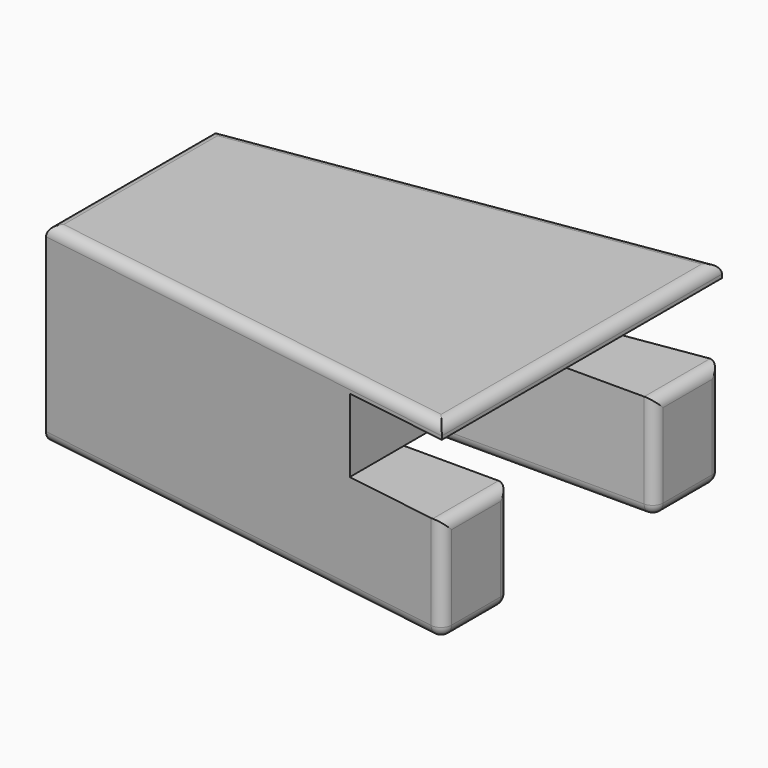
from build123d import *

# Parameters (mm, degrees)
F0_W         = 64.5
F0_H         = 13
F0_H_2       = 2
F1_DEPTH     = 12.5
F2_DEPTH     = 15
F4_DEPTH     = 15
F6_T1_DEPTH  = 72.7705906209
F6_T3_DEPTH  = 57.5
F6_T5_DEPTH  = 72.7705906209
F6_T7_DEPTH  = 37.5
F6_T9_DEPTH  = 66.75
F6_T11_DEPTH = 67.2701117692
F6_T13_DEPTH = 8.7495211484
F6_T15_DEPTH = 67.2701117692
F6_T17_DEPTH = 8.7495211484
F6_T19_DEPTH = 17.8761971291
F6_T21_DEPTH = 17.25
F6_T23_DEPTH = 19.5
F6_T25_DEPTH = 19.5
F6_S29_W     = 1.53
F6_S29_H     = 1.53
F6_T30_DEPTH = 1.53
F6_T36_DEPTH = 1.53
F6_S41_W     = 1.53
F6_S41_H     = 1.53
F6_T42_DEPTH = 1.53
F6_T48_DEPTH = 1.53
F6_T54_DEPTH = 9.5
F6_S55_R     = 1.5
F6_T56_DEPTH = 6
F6_T60_DEPTH = 9.5
F6_S61_R     = 1.5
F6_T62_DEPTH = 6
F6_T66_DEPTH = 9.5
F6_S67_R     = 1.5
F6_T68_DEPTH = 6
F6_T72_DEPTH = 9.5
F6_S73_R     = 1.5
F6_T74_DEPTH = 6


# Not quite as in the source:
# - a fillet or chamfer that OpenCascade refuses, or shapes differently, is made with other operations: its cross-section is extruded or revolved along the edge and cut away or added
# - a feature names something its author has since deleted; it is built from what else it names


with BuildPart() as f1:
    # F0 (on Top) → F1 (new body)
    with BuildSketch(Plane.XY):
        with Locations((-32.25, -6.5)):
            Rectangle(F0_W, F0_H)
        with Locations((-32.25, -14)):
            Rectangle(F0_W, F0_H_2)
        Polygon((0, -15), (-64.5, -15), (0, -25), align=None)
    extrude(amount=F1_DEPTH)

    # F0 (on Top) → F2 (join)
    with BuildSketch(Plane.XY):
        with Locations((-32.25, -14)):
            Rectangle(F0_W, F0_H_2)
        Polygon((0, -15), (-64.5, -15), (0, -25), align=None)
    extrude(amount=-F2_DEPTH)

    # F3 (on face) → F4 (cut)
    with BuildSketch(Plane.YZ):
        Polygon((-13, 0), (0, 0), (0, 10.5), (-25, 10.5), (-25, 0), align=None)
    extrude(amount=-F4_DEPTH, mode=Mode.SUBTRACT)

    # F5: F1 across plane


with BuildPart() as f1_1:
    add(f1.part)
    add(f1.part.mirror(Plane.XZ))

    # F6: fillet of radius 1.5 on 18 edges, made by hand

    # F6_s2 → F6_t1 (cut)
    with BuildSketch(Plane(origin=(-64.4207380098, 9.9877113194, 0), x_dir=(0, 0, 1), z_dir=(0.9881939076, -0.1532083578, 0))):
        with BuildLine():
            ThreePointArc((11, 24.7048476911), (12.0606601718, 24.2655078629), (12.5, 23.2048476911))
            Line((12.5, 23.2048476911), (12.5, 24.7048476911))
            Line((12.5, 24.7048476911), (11, 24.7048476911))
        make_face()
    extrude(amount=F6_T1_DEPTH, mode=Mode.SUBTRACT)

    # F6_s4 → F6_t3 (cut)
    with BuildSketch(Plane.XZ.offset(-28.75)):
        with BuildLine():
            ThreePointArc((-1.5, 12.5), (-0.4393398282, 12.0606601718), (0, 11))
            Line((0, 11), (0, 12.5))
            Line((0, 12.5), (-1.5, 12.5))
        make_face()
    extrude(amount=F6_T3_DEPTH, mode=Mode.SUBTRACT)

    # F6_s6 → F6_t5 (cut)
    with BuildSketch(Plane(origin=(-64.4207380098, -9.9877113194, 0), x_dir=(0, 0, 1), z_dir=(0.9881939076, 0.1532083578, 0))):
        with BuildLine():
            ThreePointArc((12.5, -23.2048476911), (12.0606601718, -24.2655078629), (11, -24.7048476911))
            Line((11, -24.7048476911), (12.5, -24.7048476911))
            Line((12.5, -24.7048476911), (12.5, -23.2048476911))
        make_face()
    extrude(amount=F6_T5_DEPTH, mode=Mode.SUBTRACT)

    # F6_s8 → F6_t7 (cut)
    with BuildSketch(Plane.XZ.offset(-18.75)):
        with BuildLine():
            ThreePointArc((-63, 12.5), (-64.0606601718, 12.0606601718), (-64.5, 11))
            Line((-64.5, 11), (-64.5, 12.5))
            Line((-64.5, 12.5), (-63, 12.5))
        make_face()
    extrude(amount=F6_T7_DEPTH, mode=Mode.SUBTRACT)

    # F6_s10 → F6_t9 (cut)
    with BuildSketch(Plane.YZ.offset(-68.25)):
        with BuildLine():
            ThreePointArc((-13, -13.5), (-13.4393398282, -14.5606601718), (-14.5, -15))
            Line((-14.5, -15), (-13, -15))
            Line((-13, -15), (-13, -13.5))
        make_face()
        with BuildLine():
            ThreePointArc((13, -13.5), (13.4393398282, -14.5606601718), (14.5, -15))
            Line((14.5, -15), (13, -15))
            Line((13, -15), (13, -13.5))
        make_face()
    extrude(amount=F6_T9_DEPTH, mode=Mode.SUBTRACT)

    # F6_s12 → F6_t11 (cut)
    with BuildSketch(Plane(origin=(-64.4207380098, 9.9877113194, 0), x_dir=(0, 0, 1), z_dir=(0.9881939076, -0.1532083578, 0))):
        with BuildLine():
            ThreePointArc((-13.5, 24.7048476911), (-14.5606601718, 24.2655078629), (-15, 23.2048476911))
            Line((-15, 23.2048476911), (-15, 24.7048476911))
            Line((-15, 24.7048476911), (-13.5, 24.7048476911))
        make_face()
    extrude(amount=F6_T11_DEPTH, mode=Mode.SUBTRACT)

    # F6_s14 → F6_t13 (cut)
    with BuildSketch(Plane.XZ.offset(14.5)):
        with BuildLine():
            ThreePointArc((0, -13.5), (-0.4393398282, -14.5606601718), (-1.5, -15))
            Line((-1.5, -15), (0, -15))
            Line((0, -15), (0, -13.5))
        make_face()
    extrude(amount=F6_T13_DEPTH, mode=Mode.SUBTRACT)

    # F6_s16 → F6_t15 (cut)
    with BuildSketch(Plane(origin=(-64.4207380098, -9.9877113194, 0), x_dir=(0, 0, 1), z_dir=(0.9881939076, 0.1532083578, 0))):
        with BuildLine():
            ThreePointArc((-15, -23.2048476911), (-14.5606601718, -24.2655078629), (-13.5, -24.7048476911))
            Line((-13.5, -24.7048476911), (-15, -24.7048476911))
            Line((-15, -24.7048476911), (-15, -23.2048476911))
        make_face()
    extrude(amount=F6_T15_DEPTH, mode=Mode.SUBTRACT)

    # F6_s18 → F6_t17 (cut)
    with BuildSketch(Plane.XZ.offset(-23.2495211484)):
        with BuildLine():
            ThreePointArc((-1.5, -15), (-0.4393398282, -14.5606601718), (0, -13.5))
            Line((0, -13.5), (0, -15))
            Line((0, -15), (-1.5, -15))
        make_face()
    extrude(amount=F6_T17_DEPTH, mode=Mode.SUBTRACT)

    # F6_s20 → F6_t19 (cut)
    with BuildSketch(Plane.XY.offset(-13.5)):
        with BuildLine():
            ThreePointArc((-1.7298125367, -24.7318120098), (-0.5239669076, -24.3885380062), (0, -23.2495211484))
            Line((0, -23.2495211484), (0, -25))
            Line((0, -25), (-1.7298125367, -24.7318120098))
        make_face()
        with BuildLine():
            ThreePointArc((0, 23.2495211484), (-0.5239669076, 24.3885380062), (-1.7298125367, 24.7318120098))
            Line((-1.7298125367, 24.7318120098), (0, 25))
            Line((0, 25), (0, 23.2495211484))
        make_face()
    extrude(amount=F6_T19_DEPTH, mode=Mode.SUBTRACT)

    # F6_s22 → F6_t21 (cut)
    with BuildSketch(Plane.XY.offset(-13.5)):
        with BuildLine():
            ThreePointArc((-1.5, -13), (-0.4393398282, -13.4393398282), (0, -14.5))
            Line((0, -14.5), (0, -13))
            Line((0, -13), (-1.5, -13))
        make_face()
        with BuildLine():
            ThreePointArc((-1.5, 13), (-0.4393398282, 13.4393398282), (0, 14.5))
            Line((0, 14.5), (0, 13))
            Line((0, 13), (-1.5, 13))
        make_face()
    extrude(amount=F6_T21_DEPTH, mode=Mode.SUBTRACT)

    # F6_s24 → F6_t23 (cut)
    with BuildSketch(Plane.XZ.offset(9.25)):
        with BuildLine():
            ThreePointArc((-1.5, 0), (-0.4393398282, -0.4393398282), (0, -1.5))
            Line((0, -1.5), (0, 0))
            Line((0, 0), (-1.5, 0))
        make_face()
    extrude(amount=F6_T23_DEPTH, mode=Mode.SUBTRACT)

    # F6_s26 → F6_t25 (cut)
    with BuildSketch(Plane.XZ.offset(-28.75)):
        with BuildLine():
            ThreePointArc((-1.5, 0), (-0.4393398282, -0.4393398282), (0, -1.5))
            Line((0, -1.5), (0, 0))
            Line((0, 0), (-1.5, 0))
        make_face()
    extrude(amount=F6_T25_DEPTH, mode=Mode.SUBTRACT)


with BuildPart() as f6_tool28:
    # F6_s29 → F6_t30 (new body)
    with BuildSketch(Plane.YZ.offset(-1.5)):
        with Locations((-13.735, -14.265)):
            Rectangle(F6_S29_W, F6_S29_H)
    extrude(amount=F6_T30_DEPTH)

    # F6_s31 → F6_t32 (revolve, cut)
    with BuildSketch(Plane(origin=(-1.5, -14.5, -13.5), x_dir=(0, -0.7071067812, 0.7071067812), z_dir=(0, 0.7071067812, 0.7071067812))):
        with BuildLine():
            ThreePointArc((0, -1.5), (1.5, 0), (0, 1.5))
            Line((0, 1.5), (0, -1.5))
        make_face()
    revolve(axis=Axis((-1.5, -14.5, -13.5), (1, 0, 0)), mode=Mode.SUBTRACT)


with BuildPart() as f1_2:
    add(f1_1.part)

    # F6_t27: cut F6_tool28
    add(f6_tool28.part, mode=Mode.SUBTRACT)


with BuildPart() as f6_tool34:
    # F6_s35 → F6_t36 (new body)
    with BuildSketch(Plane.XY.offset(-13.5)):
        Polygon((-1.5, -23.2495211484), (-1.7344087874, -24.761457827), (0.03, -25.035009577), (0.03, -23.2495211484), align=None)
    extrude(amount=-F6_T36_DEPTH)

    # F6_s37 → F6_t38 (revolve, cut)
    with BuildSketch(Plane(origin=(-1.5, -23.2495211484, -13.5), x_dir=(-0.6506887283, 0.7593445719, 0), z_dir=(-0.7593445719, -0.6506887283, 0))):
        with BuildLine():
            ThreePointArc((0, -1.5), (1.5, 0), (0, 1.5))
            Line((0, 1.5), (0, -1.5))
        make_face()
    revolve(axis=Axis((-1.5, -23.2495211484, -13.5), (0, 0, -1)), mode=Mode.SUBTRACT)


with BuildPart() as f1_3:
    add(f1_2.part)

    # F6_t33: cut F6_tool34
    add(f6_tool34.part, mode=Mode.SUBTRACT)


with BuildPart() as f6_tool40:
    # F6_s41 → F6_t42 (new body)
    with BuildSketch(Plane.YZ.offset(-1.5)):
        with Locations((13.735, -14.265)):
            Rectangle(F6_S41_W, F6_S41_H)
    extrude(amount=F6_T42_DEPTH)

    # F6_s43 → F6_t44 (revolve, cut)
    with BuildSketch(Plane(origin=(-1.5, 14.5, -13.5), x_dir=(0, 0.7071067812, 0.7071067812), z_dir=(0, 0.7071067812, -0.7071067812))):
        with BuildLine():
            ThreePointArc((0, -1.5), (1.5, 0), (0, 1.5))
            Line((0, 1.5), (0, -1.5))
        make_face()
    revolve(axis=Axis((-1.5, 14.5, -13.5), (1, 0, 0)), mode=Mode.SUBTRACT)


with BuildPart() as f1_4:
    add(f1_3.part)

    # F6_t39: cut F6_tool40
    add(f6_tool40.part, mode=Mode.SUBTRACT)


with BuildPart() as f6_tool46:
    # F6_s47 → F6_t48 (new body)
    with BuildSketch(Plane.XY.offset(-13.5)):
        Polygon((-1.5, 23.2495211484), (0.03, 23.2495211484), (0.03, 25.035009577), (-1.7344087874, 24.761457827), align=None)
    extrude(amount=-F6_T48_DEPTH)

    # F6_s49 → F6_t50 (revolve, cut)
    with BuildSketch(Plane(origin=(-1.5, 23.2495211484, -13.5), x_dir=(-0.6506887283, -0.7593445719, 0), z_dir=(0.7593445719, -0.6506887283, 0))):
        with BuildLine():
            ThreePointArc((0, -1.5), (1.5, 0), (0, 1.5))
            Line((0, 1.5), (0, -1.5))
        make_face()
    revolve(axis=Axis((-1.5, 23.2495211484, -13.5), (0, 0, -1)), mode=Mode.SUBTRACT)


with BuildPart() as f1_5:
    add(f1_4.part)

    # F6_t45: cut F6_tool46
    add(f6_tool46.part, mode=Mode.SUBTRACT)


with BuildPart() as f6_tool52:
    # F6_s53 → F6_t54 (new body)
    with BuildSketch(Plane.XZ.offset(9.25)):
        with BuildLine():
            ThreePointArc((-63, -15), (-64.0606601718, -14.5606601718), (-64.5, -13.5))
            Line((-64.5, -13.5), (-64.5, -15))
            Line((-64.5, -15), (-63, -15))
        make_face()
    extrude(amount=F6_T54_DEPTH)

    # F6_s55 → F6_t56 (cut, symmetric)
    with BuildSketch(Plane(origin=(-60.1810089756, 9.3303889885, 0), x_dir=(0, 0, 1), z_dir=(-0.9881939076, 0.1532083578, 0))):
        with Locations((-13.5, -23.2048476911)):
            Circle(F6_S55_R)
    extrude(amount=F6_T56_DEPTH, both=True, mode=Mode.SUBTRACT)


with BuildPart() as f1_6:
    add(f1_5.part)

    # F6_t51: cut F6_tool52
    add(f6_tool52.part, mode=Mode.SUBTRACT)


with BuildPart() as f6_tool58:
    # F6_s59 → F6_t60 (new body)
    with BuildSketch(Plane.XZ.offset(9.25)):
        with BuildLine():
            ThreePointArc((-63, -15), (-64.0606601718, -14.5606601718), (-64.5, -13.5))
            Line((-64.5, -13.5), (-64.5, -15))
            Line((-64.5, -15), (-63, -15))
        make_face()
    extrude(amount=F6_T60_DEPTH)

    # F6_s61 → F6_t62 (cut, symmetric)
    with BuildSketch(Plane.YZ.offset(-63.8)):
        with Locations((-14.5, -13.5)):
            Circle(F6_S61_R)
    extrude(amount=F6_T62_DEPTH, both=True, mode=Mode.SUBTRACT)


with BuildPart() as f1_7:
    add(f1_6.part)

    # F6_t57: cut F6_tool58
    add(f6_tool58.part, mode=Mode.SUBTRACT)


with BuildPart() as f6_tool64:
    # F6_s65 → F6_t66 (new body)
    with BuildSketch(Plane.XZ.offset(-9.25)):
        with BuildLine():
            ThreePointArc((-63, -15), (-64.0606601718, -14.5606601718), (-64.5, -13.5))
            Line((-64.5, -13.5), (-64.5, -15))
            Line((-64.5, -15), (-63, -15))
        make_face()
    extrude(amount=-F6_T66_DEPTH)

    # F6_s67 → F6_t68 (cut, symmetric)
    with BuildSketch(Plane(origin=(-60.1810089756, -9.3303889885, 0), x_dir=(0, 0, 1), z_dir=(-0.9881939076, -0.1532083578, 0))):
        with Locations((-13.5, 23.2048476911)):
            Circle(F6_S67_R)
    extrude(amount=F6_T68_DEPTH, both=True, mode=Mode.SUBTRACT)


with BuildPart() as f1_8:
    add(f1_7.part)

    # F6_t63: cut F6_tool64
    add(f6_tool64.part, mode=Mode.SUBTRACT)


with BuildPart() as f6_tool70:
    # F6_s71 → F6_t72 (new body)
    with BuildSketch(Plane.XZ.offset(-9.25)):
        with BuildLine():
            ThreePointArc((-63, -15), (-64.0606601718, -14.5606601718), (-64.5, -13.5))
            Line((-64.5, -13.5), (-64.5, -15))
            Line((-64.5, -15), (-63, -15))
        make_face()
    extrude(amount=-F6_T72_DEPTH)

    # F6_s73 → F6_t74 (cut, symmetric)
    with BuildSketch(Plane.YZ.offset(-63.8)):
        with Locations((14.5, -13.5)):
            Circle(F6_S73_R)
    extrude(amount=F6_T74_DEPTH, both=True, mode=Mode.SUBTRACT)


with BuildPart() as f1_9:
    add(f1_8.part)

    # F6_t69: cut F6_tool70
    add(f6_tool70.part, mode=Mode.SUBTRACT)


solid = f1_9.part
